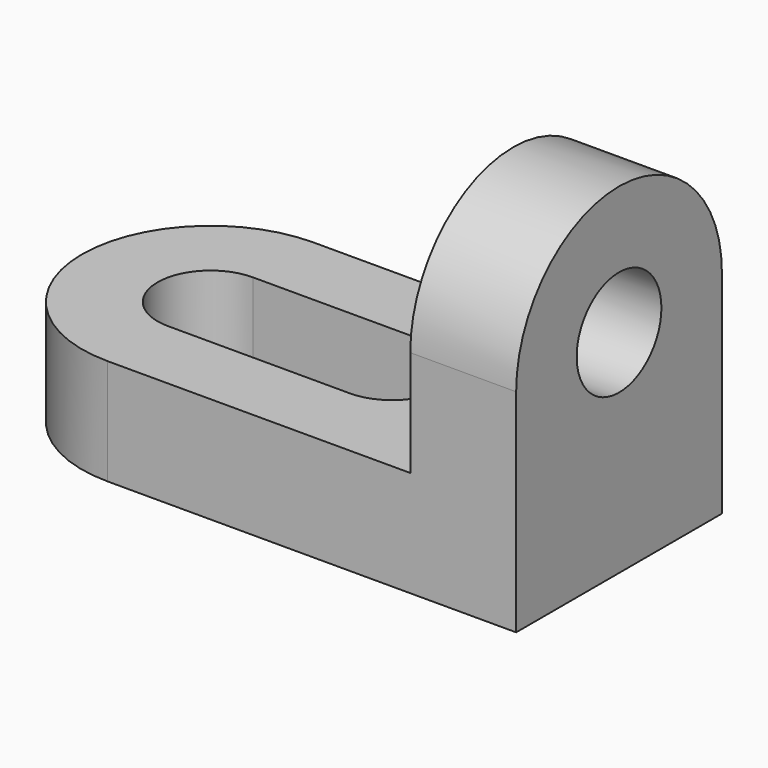
from build123d import *

# Parameters (mm, degrees)
F0_W      = 54
F0_H      = 34
F1_DEPTH  = 14
F2_W      = 14
F2_H      = 34
F3_DEPTH  = 14
F5_DEPTH  = 14
F7_DEPTH  = 14
F8_R      = 7
F9_DEPTH  = 25
F11_DEPTH = 25


with BuildPart() as f1:
    # F0 (on Top) → F1 (new body)
    with BuildSketch(Plane.XY):
        with Locations((-1.2663472444, 3.4664713239)):
            Rectangle(F0_W, F0_H)
    extrude(amount=F1_DEPTH)

    # F2 (on face) → F3 (join)
    with BuildSketch(Plane.XY.offset(14)):
        with Locations((18.7336527556, 3.4664713239)):
            Rectangle(F2_W, F2_H)
    extrude(amount=F3_DEPTH)

    # F4 (on face) → F5 (join)
    with BuildSketch(Plane.YZ.offset(25.7336527556)):
        with BuildLine():
            Line((-13.5335286761, 28), (20.4664713239, 28))
            ThreePointArc((20.4664713239, 28), (3.4664713239, 45), (-13.5335286761, 28))
        make_face()
        with BuildLine():
            ThreePointArc((-13.5335286761, 28), (3.4664713239, 11), (20.4664713239, 28))
            Line((20.4664713239, 28), (-13.5335286761, 28))
        make_face()
    extrude(amount=-F5_DEPTH)

    # F6 (on face) → F7 (join)
    with BuildSketch(Plane.XY.offset(14)):
        with BuildLine():
            Line((-28.2663472444, -13.5335286761), (-28.2663472444, 20.4664713239))
            ThreePointArc((-28.2663472444, 20.4664713239), (-45.2663472444, 3.4664713239), (-28.2663472444, -13.5335286761))
        make_face()
    extrude(amount=-F7_DEPTH)

    # F8 (on face) → F9 (cut)
    with BuildSketch(Plane.YZ.offset(25.7336527556)):
        with Locations((3.4664713239, 28)):
            Circle(F8_R)
    extrude(amount=-F9_DEPTH, mode=Mode.SUBTRACT)

    # F10 (on face) → F11 (cut)
    with BuildSketch(Plane.XY.offset(14)):
        with BuildLine():
            ThreePointArc((-27.9110185812, -3.5245043978), (-23.1925271529, -1.3560124427), (-21.2663472444, 3.4664713239))
            ThreePointArc((-21.2663472444, 3.4664713239), (-23.3165997761, 8.4162187922), (-28.2663472444, 10.4664713239))
            ThreePointArc((-28.2663472444, 10.4664713239), (-35.2640908111, 3.2887497041), (-27.9110185812, -3.5245043978))
        make_face()
        with BuildLine():
            ThreePointArc((-28.2663472444, 10.4664713239), (-23.3165997761, 8.4162187922), (-21.2663472444, 3.4664713239))
            ThreePointArc((-21.2663472444, 3.4664713239), (-23.1925271529, -1.3560124427), (-27.9110185812, -3.5245043978))
            Line((-27.9110185812, -3.5245043978), (-4.2690190308, -3.5335281663))
            ThreePointArc((-4.2690190308, -3.5335281663), (-11.2663471169, 3.4678072171), (-4.2663472444, 10.4664713239))
            Line((-4.2663472444, 10.4664713239), (-28.2663472444, 10.4664713239))
        make_face()
        with BuildLine():
            ThreePointArc((2.7336527556, 3.4664713239), (0.6834002239, 8.4162187922), (-4.2663472444, 10.4664713239))
            ThreePointArc((-4.2663472444, 10.4664713239), (-11.2663471169, 3.4678072171), (-4.2690190308, -3.5335281663))
            ThreePointArc((-4.2690190308, -3.5335281663), (0.6824555146, -1.4842206735), (2.7336527556, 3.4664713239))
        make_face()
    extrude(amount=-F11_DEPTH, mode=Mode.SUBTRACT)


solid = f1.part
